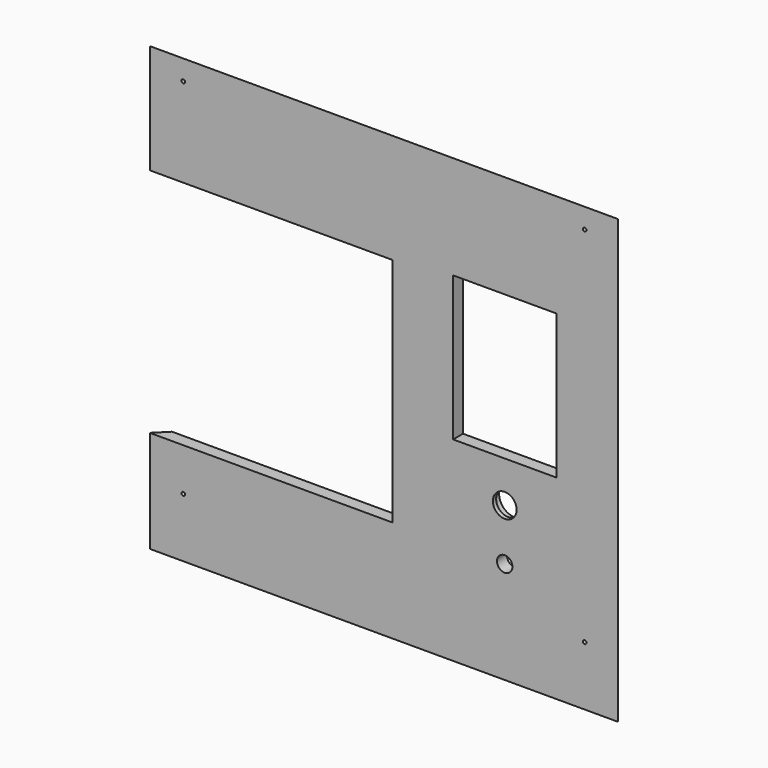
from build123d import *

# Parameters (mm, degrees)
F0_W     = 454
F0_H     = 429
F1_DEPTH = 12
F2_SIZE  = 11.99999
F3_W     = 235
F3_H     = 224
F3_W_2   = 100
F3_H_2   = 140
F3_R     = 11.5
F3_R_2   = 7.5
F4_DEPTH = 25
F6_D     = 3.5
F7_R     = 15
F7_R_2   = 11.5
F8_DEPTH = 8


# Not quite as in the source:
# - a fillet or chamfer is up to 0.001 mm smaller than in the source, because OpenCascade refuses the exact size


with BuildPart() as f1:
    # F0 (on Front) → F1 (new body)
    with BuildSketch(Plane.XZ):
        Rectangle(F0_W, F0_H)
    extrude(amount=F1_DEPTH)

    # F2 (size 12 in the source; OpenCascade refuses exactly that, so slightly less here)
    f2_edges = [f1.edges().sort_by_distance(p)[0] for p in [
        (227, 0, 0),
        (-227, 0, 0),
        (0, 0, 214.5),
    ]]
    chamfer(f2_edges, length=F2_SIZE)

    # F3 (on face) → F4 (cut)
    with BuildSketch(Plane.XZ.offset(12)):
        with Locations((-109.5, -3.5)):
            Rectangle(F3_W, F3_H)
        with Locations((117, 44.5)):
            Rectangle(F3_W_2, F3_H_2)
        with Locations((117, -65.5)):
            Circle(F3_R)
        with Locations((117, -115.5)):
            Circle(F3_R_2)
    extrude(amount=-F4_DEPTH, mode=Mode.SUBTRACT)

    # F6 (through all)
    with Locations(Plane.XZ.offset(12)):
        with Locations((-194.5, 195), (194.5, 195), (194.5, -157), (-194.5, -157)):
            Hole(F6_D / 2)

    # F7 (on face) → F8 (cut)
    with BuildSketch(Plane(origin=(0, 0, 0), x_dir=(-1, 0, 0), z_dir=(0, 1, 0))):
        with Locations((-117, -65.5)):
            Circle(F7_R)
        with Locations((-117, -65.5)):
            Circle(F7_R_2, mode=Mode.SUBTRACT)
    extrude(amount=-F8_DEPTH, mode=Mode.SUBTRACT)


solid = f1.part
